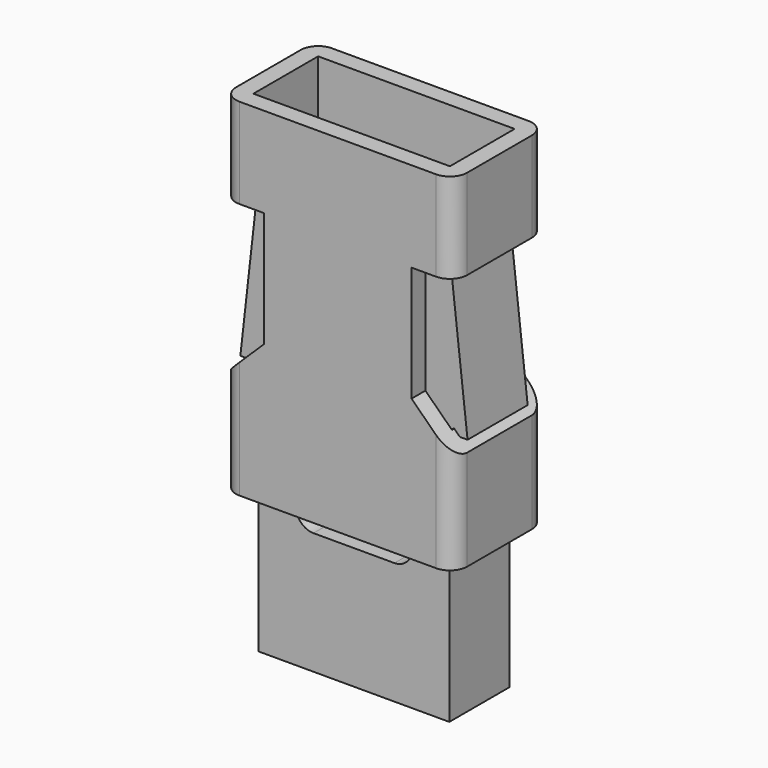
from build123d import *

# Parameters (mm, degrees)
F0_W      = 34
F0_H      = 14
F1_DEPTH  = 60
F3_DEPTH  = 12.5
F4_W      = 33
F4_H      = 13
F5_DEPTH  = 47
F6_DEPTH  = 25
F8_DEPTH  = 13
F9_W      = 10.0071702135
F9_H      = 7.5427786708
F10_DEPTH = 13
F11_R     = 3
F12_SIZE  = 0.5


with BuildPart() as f1:
    # F0 (on Top) → F1 (new body)
    with BuildSketch(Plane.XY):
        with BuildLine():
            Line((-17, -10), (17, -10))
            ThreePointArc((17, -10), (19.1213203436, -9.1213203436), (20, -7))
            Line((20, -7), (20, 7))
            ThreePointArc((20, 7), (19.1213203436, 9.1213203436), (17, 10))
            Line((17, 10), (-17, 10))
            ThreePointArc((-17, 10), (-19.1213203436, 9.1213203436), (-20, 7))
            Line((-20, 7), (-20, -7))
            ThreePointArc((-20, -7), (-19.1213203436, -9.1213203436), (-17, -10))
        make_face()
        Rectangle(F0_W, F0_H, mode=Mode.SUBTRACT)
    extrude(amount=F1_DEPTH)

    # F2 (on Front) → F3 (cut, symmetric)
    with BuildSketch(Plane.XZ):
        Polygon((-25.0430125743, 44.4069132209), (-22.8498019278, 14.5792569965), (-12.7610368654, 24.4487021118), (-12.7610368654, 44.4069132209), align=None)
        Polygon((22.8498019278, 14.5792569965), (25.0430125743, 44.4069132209), (12.7610368654, 44.4069132209), (12.7610368654, 24.4487021118), align=None)
    extrude(amount=F3_DEPTH, both=True, mode=Mode.SUBTRACT)

    # F12
    f12_edges = [f1.edges().sort_by_distance(p)[0] for p in [
        (17, 0, 20.30189),
        (-17, 0, 20.30189),
    ]]
    chamfer(f12_edges, length=F12_SIZE)


with BuildPart() as f5:
    # F4 (on face) → F5 (new body)
    with BuildSketch(Plane(origin=(0, 0, 0), x_dir=(1, 0, 0), z_dir=(0, 0, -1))):
        Rectangle(F4_W, F4_H)
    extrude(amount=-F5_DEPTH)

    # F6 (add): a face of the model
    f6_faces = [f5.faces().sort_by_distance(p)[0] for p in [
        (0, 0, 0),
    ]]
    extrude(f6_faces, amount=F6_DEPTH)

    # F7 (on face) → F8 (join, through all)
    with BuildSketch(Plane.XZ.offset(6.5)):
        Polygon((-16.5, 19), (-16.5, 47), (-19.6545496583, 19), align=None)
        Polygon((19.6545496583, 19), (16.5, 47), (16.5, 19), align=None)
    extrude(amount=-F8_DEPTH)

    # F9 (on face) → F10 (cut, through all)
    with BuildSketch(Plane.XZ.offset(6.5)):
        Polygon((-10.0071702135, 47), (-10.0071702135, 19), (-10.0071702135, -3.8913467145), (0, -3.8913467145), (0, 47), align=None)
        with Locations((-5.0035851068, 50.7713893354)):
            Rectangle(F9_W, F9_H)
        with Locations((5.0035851068, 50.7713893354)):
            Rectangle(F9_W, F9_H)
        Polygon((0, 47), (0, -3.8913467145), (10.0071702135, -3.8913467145), (10.0071702135, 19), (10.0071702135, 47), align=None)
    extrude(amount=-F10_DEPTH, mode=Mode.SUBTRACT)

    # F11
    f11_edges = [f5.edges().sort_by_distance(p)[0] for p in [
        (16.5, 0, 47),
        (-16.5, 0, 47),
        (-10.00717, 0, -3.891347),
        (10.00717, 0, -3.891347),
        (10.00717, 0, 47),
        (-10.00717, 0, 47),
    ]]
    fillet(f11_edges, radius=F11_R)


solid = Compound([f1.part, f5.part])
